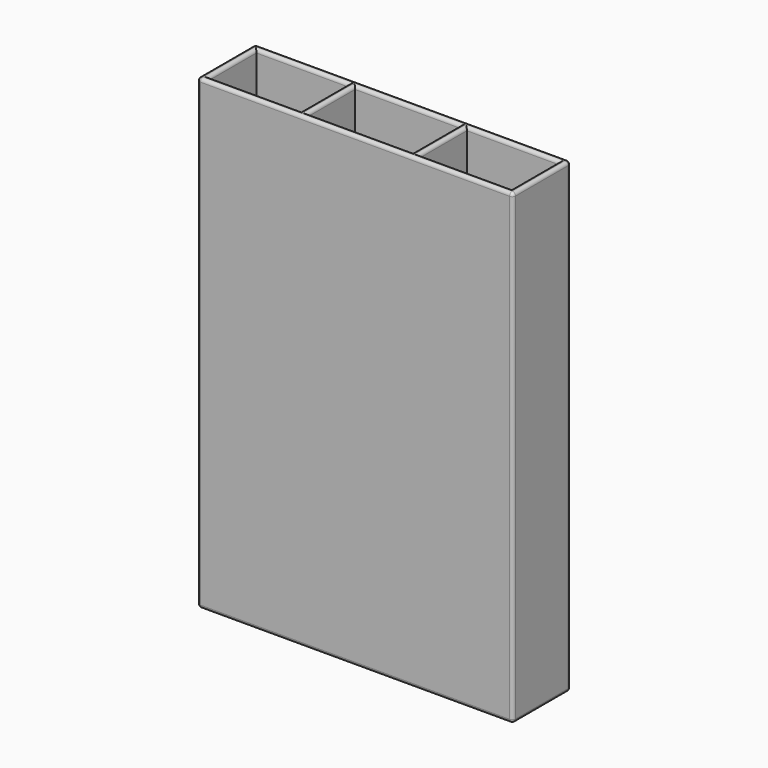
from build123d import *

# Parameters (mm, degrees)
F0_W     = 14
F0_H     = 9
F0_W_2   = 1
F0_W_3   = 16
F1_DEPTH = 1
F0_W_4   = 48
F0_H_2   = 11
F2_DEPTH = 71
F3_DEPTH = 71
F4_R     = 0.49999


# Not quite as in the source:
# - a fillet or chamfer is up to 0.001 mm smaller than in the source, because OpenCascade refuses the exact size


with BuildPart() as f1:
    # F0 (on Top) → F1 (new body)
    with BuildSketch(Plane.XY):
        with Locations((-11.0720558167, 5.5)):
            Rectangle(F0_W, F0_H)
        with Locations((-3.5720558167, 5.5)):
            Rectangle(F0_W_2, F0_H)
        with Locations((4.9279441833, 5.5)):
            Rectangle(F0_W_3, F0_H)
        with Locations((13.4279441833, 5.5)):
            Rectangle(F0_W_2, F0_H)
        with Locations((20.9279441833, 5.5)):
            Rectangle(F0_W, F0_H)
    extrude(amount=F1_DEPTH)

    # F0 (on Top) → F2 (join)
    with BuildSketch(Plane.XY):
        with Locations((4.9279441833, 5.5)):
            Rectangle(F0_W_4, F0_H_2)
        Polygon((-18.0720558167, 1), (-18.0720558167, 10), (-4.0720558167, 10), (-3.0720558167, 10), (12.9279441833, 10), (13.9279441833, 10), (27.9279441833, 10), (27.9279441833, 1), (13.9279441833, 1), (12.9279441833, 1), (-3.0720558167, 1), (-4.0720558167, 1), align=None, mode=Mode.SUBTRACT)
    extrude(amount=F2_DEPTH)

    # F0 (on Top) → F3 (join)
    with BuildSketch(Plane.XY):
        with Locations((-3.5720558167, 5.5)):
            Rectangle(F0_W_2, F0_H)
        with Locations((13.4279441833, 5.5)):
            Rectangle(F0_W_2, F0_H)
    extrude(amount=F3_DEPTH)

    # F4 (radius 0.5 in the source; OpenCascade refuses exactly that, so slightly less here)
    f4_edges = [f1.edges().sort_by_distance(p)[0] for p in [
        (-19.072056, 5.5, 71),
        (4.927944, 0, 71),
        (28.927944, 5.5, 71),
        (4.927944, 11, 71),
        (-18.072056, 5.5, 71),
        (-11.072056, 10, 71),
        (-4.072056, 5.5, 71),
        (-11.072056, 1, 71),
        (20.927944, 10, 71),
        (27.927944, 5.5, 71),
        (20.927944, 1, 71),
        (13.927944, 5.5, 71),
        (4.927944, 10, 71),
        (12.927944, 5.5, 71),
        (4.927944, 1, 71),
        (-3.072056, 5.5, 71),
        (28.927944, 11, 35.5),
        (-19.072056, 11, 35.5),
        (4.927944, 11, 0),
        (-19.072056, 0, 35.5),
        (-19.072056, 5.5, 0),
        (28.927944, 0, 35.5),
        (4.927944, 0, 0),
        (28.927944, 5.5, 0),
    ]]
    fillet(f4_edges, radius=F4_R)


solid = f1.part
